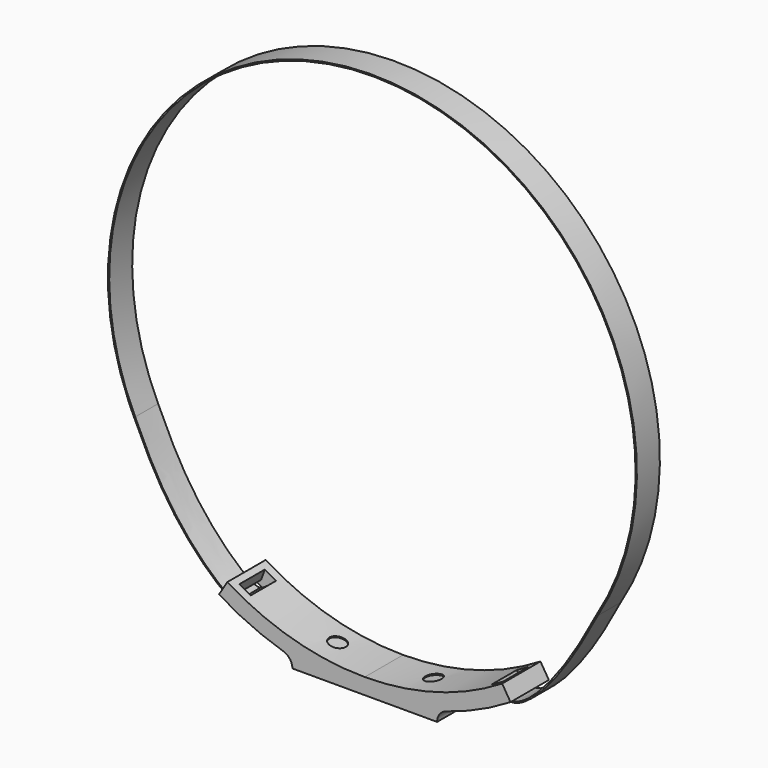
from build123d import *

# Parameters (mm, degrees)
F1_DEPTH     = 19.05
F3_D         = 6.5278
F3_DEPTH     = 101.6
F3_TIP       = 1.9611489744
F7_DEPTH     = 25.4
F9_DEPTH     = 25.4
F10_T1_DEPTH = 12.7
F11_T4_DEPTH = 19.05
F11_T9_DEPTH = 19.05
F13_START    = -3.81
F13_DEPTH    = 11.43


# Not quite as in the source:
# - a fillet or chamfer that OpenCascade refuses, or shapes differently, is made with other operations: its cross-section is extruded or revolved along the edge and cut away or added
# - ends of sketch curves that miss each other by under 0.0002 mm in the source are joined
# - the dataset's text gives a spline's control points without its knots; the knots are read off the source's solid


with BuildPart() as f1:
    # F0 (on Front) → F1 (new body)
    with BuildSketch(Plane.XZ):
        with BuildLine():
            Line((0, 0.9525), (28.7734375, 0.9525))
            Line((28.7734375, 0.9525), (28.7734375, 4.7648106998))
            ThreePointArc((28.7734375, 4.7648106998), (43.8235256978, 10.0149953703), (57.9615735284, 17.3760548981))
            Line((57.9615735284, 17.3760548981), (54.630448613, 22.7821724327))
            ThreePointArc((54.630448613, 22.7821724327), (28.390606608, 11.2471255737), (0, 7.3025))
            ThreePointArc((0, 7.3025), (-28.390606608, 11.2471255737), (-54.630448613, 22.7821724327))
            Line((-54.630448613, 22.7821724327), (-57.9615735284, 17.3760548981))
            ThreePointArc((-57.9615735284, 17.3760548981), (-43.8235256978, 10.0149953703), (-28.7734375, 4.7648106998))
            Line((-28.7734375, 4.7648106998), (-28.7734375, 0.9525))
            Line((-28.7734375, 0.9525), (0, 0.9525))
        make_face()
    extrude(amount=F1_DEPTH)

    # F3
    with Locations(Plane(origin=(0, 0, 0.9525), x_dir=(1, 0, 0), z_dir=(0, 0, -1))):
        with Locations((-19.05, 8.706397377), (19.05, 8.706397377)):
            Hole(F3_D / 2, depth=F3_DEPTH)
            with Locations((0, 0, -(F3_DEPTH + F3_TIP / 2))):  # 118° drill point
                Cone(0, F3_D / 2, F3_TIP, mode=Mode.SUBTRACT)

    # F6 (on face) → F7 (cut)
    with BuildSketch(Plane(origin=(0.9315005668, 0, 2.5592767734), x_dir=(0.9396926208, 0, -0.3420201433), z_dir=(0.3420201433, 0, 0.9396926208))):
        Polygon((-56.5877913126, -15.875), (-51.5077913126, -15.875), (-51.5077913126, -3.175), (-56.5877913126, -3.175), (-56.5877913126, -9.525), align=None)
    extrude(amount=-F7_DEPTH, mode=Mode.SUBTRACT)

    # F8 (on face) → F9 (cut)
    with BuildSketch(Plane(origin=(-0.9315005668, 0, 2.5592767734), x_dir=(0.9396926208, 0, 0.3420201433), z_dir=(-0.3420201433, 0, 0.9396926208))):
        Polygon((56.5877913126, -9.525), (56.5877913126, -3.175), (51.5077913126, -3.175), (51.5077913126, -15.875), (56.5877913126, -15.875), align=None)
    extrude(amount=-F9_DEPTH, mode=Mode.SUBTRACT)

    # F10: chamfer of 2.032 on 2 edges, made by hand

    # F10_s2 → F10_t1 (cut)
    with BuildSketch(Plane.XZ.offset(3.175)):
        with BuildLine():
            Line((-56.4802385277, 16.4064101357), (-53.8380025429, 17.3499641227))
            Line((-53.8380025429, 17.3499641227), (-53.7998134348, 17.3360644241))
            ThreePointArc((-53.7998134348, 17.3360644241), (-54.2182847726, 16.36929669), (-54.5779497805, 15.3811252023))
            Line((-54.5779497805, 15.3811252023), (-54.6362275834, 15.359697094))
            ThreePointArc((-54.6362275834, 15.359697094), (-55.5554397743, 15.8882458284), (-56.5009847135, 16.3714643867))
            Line((-56.5009847135, 16.3714643867), (-56.4802385277, 16.4064101357))
        make_face()
        with BuildLine():
            Line((56.4802385277, 16.4064101357), (53.8380025429, 17.3499641227))
            Line((53.8380025429, 17.3499641227), (53.7998134348, 17.3360644241))
            ThreePointArc((53.7998134348, 17.3360644241), (54.2182847726, 16.36929669), (54.5779497805, 15.3811252023))
            Line((54.5779497805, 15.3811252023), (54.6362275834, 15.359697094))
            ThreePointArc((54.6362275834, 15.359697094), (55.5554397743, 15.8882458284), (56.5009847135, 16.3714643867))
            Line((56.5009847135, 16.3714643867), (56.4802385277, 16.4064101357))
        make_face()
    extrude(amount=F10_T1_DEPTH, mode=Mode.SUBTRACT)

    # F11: fillet of radius 5.08 on 2 edges, made by hand


with BuildPart() as f11_tool2:
    # F11_s3 → F11_t4 (new body)
    with BuildSketch(Plane.XZ):
        with BuildLine():
            ThreePointArc((32.3653743132, 5.7991251695), (29.7689692978, 3.9624749409), (28.7734375, 0.9419585107))
            Line((28.7734375, 0.9419585107), (28.7734375, 4.7648106998))
            ThreePointArc((28.7734375, 4.7648106998), (30.5737800916, 5.266777394), (32.3653743132, 5.7991251695))
        make_face()
    extrude(amount=F11_T4_DEPTH)

    split(bisect_by=Plane.XY.offset(0.9525), keep=Keep.TOP)


with BuildPart() as f1_1:
    add(f1.part)

    # F11_t1: union F11_tool2
    add(f11_tool2.part)


with BuildPart() as f11_tool7:
    # F11_s8 → F11_t9 (new body)
    with BuildSketch(Plane.XZ):
        with BuildLine():
            ThreePointArc((-28.7734375, 0.9419585107), (-29.7689692978, 3.9624749409), (-32.3653743132, 5.7991251695))
            ThreePointArc((-32.3653743132, 5.7991251695), (-30.5737800916, 5.266777394), (-28.7734375, 4.7648106998))
            Line((-28.7734375, 4.7648106998), (-28.7734375, 0.9419585107))
        make_face()
    extrude(amount=F11_T9_DEPTH)

    split(bisect_by=Plane.XY.offset(0.9525), keep=Keep.TOP)


with BuildPart() as f1_2:
    add(f1_1.part)

    # F11_t6: union F11_tool7
    add(f11_tool7.part)


with BuildPart() as f13:
    # F12 (on face) → F13 (new body)
    with BuildSketch(Plane.XZ.offset(19.05).offset(F13_START)):
        with BuildLine():
            add(Edge.make_bspline(
                [(97.7812934658, 72.7565466816), (95.0915874954, 67.2526865805), (92.3916550741, 61.7538834708), (89.5893457762, 56.3831369507)],
                knots=[0, 0, 0, 0, 0.1467920374, 0.1467920374, 0.1467920374, 0.1467920374], degree=3))
            ThreePointArc((89.5893457762, 56.3831369507), (94.042337535, 64.3912185408), (97.7812934658, 72.7565466816))
        make_face()
        with BuildLine():
            add(Edge.make_bspline(
                [(89.112833025, 56.5680768855), (87.1535051538, 52.8143908139), (83.9230985786, 46.8814228282), (79.1843120961, 39.086281514), (75.0604811368, 32.9606078689), (70.6811123978, 27.195171834), (66.9878253233, 23.0075171537), (64.107119758, 20.212335288), (62.0108024209, 18.440572074), (60.0075643358, 17.04001445), (58.4439275603, 16.2205997367), (57.2751800485, 15.792809978), (56.447710407, 15.5904406243), (55.6612536188, 15.5025921765), (55.1398399584, 15.5086945326), (54.8758058385, 15.5283343935), (54.8530867048, 15.5301494973)],
                knots=[0.1472484928, 0.1472484928, 0.1472484928, 0.1472484928, 0.25, 0.3125, 0.375, 0.4375, 0.5, 0.53125, 0.5625, 0.59375, 0.625, 0.640625, 0.65625, 0.671875, 0.6875, 0.6889755322, 0.6889755322, 0.6889755322, 0.6889755322], degree=3))
            ThreePointArc((54.8530867048, 15.5301494973), (54.4873779941, 15.3219208334), (54.1208788351, 15.1150865908))
            add(Edge.make_bspline(
                [(89.5893457762, 56.3831369507), (85.3004601923, 48.1633029224), (75.0997889772, 30.3241377329), (60.7024662065, 14.841829536), (54.9116352389, 14.9693315987), (54.1208788351, 15.1150865908)],
                knots=[0.1467920374, 0.1467920374, 0.1467920374, 0.1467920374, 0.3714546946, 0.6528345101, 0.7032287333, 0.7032287333, 0.7032287333, 0.7032287333], degree=3))
            add(Edge.make_bspline(
                [(97.7812934658, 72.7565466816), (95.0915874954, 67.2526865805), (92.3916550741, 61.7538834708), (89.5893457762, 56.3831369507)],
                knots=[0, 0, 0, 0, 0.1467920374, 0.1467920374, 0.1467920374, 0.1467920374], degree=3))
            ThreePointArc((97.7812934658, 72.7565466816), (-1.0915815894, 216.5928342155), (-96.9570973239, 70.7349378707))
            add(Edge.make_bspline(
                [(-96.9570973239, 70.7349378707), (-96.2699684757, 69.1942721991), (-95.5817912633, 67.6542476227), (-94.885448022, 66.1155092588)],
                knots=[0, 0, 0, 0, 0.0480445963, 0.0480445963, 0.0480445963, 0.0480445963], degree=3))
            add(Edge.make_bspline(
                [(-94.885448022, 66.1155092588), (-90.0354933898, 55.3983645898), (-79.6735313167, 34.3533190654), (-57.5015516811, 13.5748962232), (-53.363721711, 14.4225193998), (-53.0698134343, 14.5320516363)],
                knots=[0.0480445963, 0.0480445963, 0.0480445963, 0.0480445963, 0.3826699627, 0.7089897606, 0.736391242, 0.736391242, 0.736391242, 0.736391242], degree=3))
            ThreePointArc((-53.0698134343, 14.5320516363), (-53.393256487, 14.7098774691), (-53.7161036897, 14.8887828038))
            add(Edge.make_bspline(
                [(-94.3249878412, 66.1093333744), (-93.2420344254, 63.7191576967), (-90.2940452977, 57.3422461891), (-85.9865677113, 49.0350531394), (-81.7231896657, 42.182614942), (-79.0480730962, 38.2922627791), (-76.9119458126, 35.3892927255), (-74.6283332446, 32.4968598043), (-71.4312912207, 28.7060070403), (-68.1062078289, 25.1211706689), (-64.8409274917, 21.9448539228), (-62.4700075431, 19.8182013503), (-60.2258045547, 17.9985331885), (-58.1591419069, 16.5377888749), (-56.6307697244, 15.663594476), (-55.5586001999, 15.1955970793), (-54.841625032, 14.9654820035), (-54.2243938183, 14.8583814899), (-53.8854699098, 14.8664131973), (-53.7237397991, 14.8877344036), (-53.7161036897, 14.8887828038)],
                knots=[0.0502911195, 0.0502911195, 0.0502911195, 0.0502911195, 0.125, 0.25, 0.3125, 0.34375, 0.375, 0.40625, 0.4375, 0.5, 0.53125, 0.5625, 0.59375, 0.625, 0.65625, 0.671875, 0.6875, 0.703125, 0.71875, 0.7195270393, 0.7195270393, 0.7195270393, 0.7195270393], degree=3))
            ThreePointArc((-94.3249878412, 66.1093333744), (5.4360404927, 215.9544649915), (89.112833025, 56.5680768855))
        make_face()
        with BuildLine():
            ThreePointArc((-96.9570973239, 70.7349378707), (-95.9490767615, 68.4127544207), (-94.885448022, 66.1155092588))
            add(Edge.make_bspline(
                [(-96.9570973239, 70.7349378707), (-96.2699684757, 69.1942721991), (-95.5817912633, 67.6542476227), (-94.885448022, 66.1155092588)],
                knots=[0, 0, 0, 0, 0.0480445963, 0.0480445963, 0.0480445963, 0.0480445963], degree=3))
        make_face()
        with BuildLine():
            ThreePointArc((54.1208788351, 15.1150865908), (54.4873779941, 15.3219208334), (54.8530867048, 15.5301494973))
            add(Edge.make_bspline(
                [(54.8530867048, 15.5301494973), (54.3946418593, 15.5667761121), (53.5078157419, 15.7423770413), (52.3566642919, 16.2141141425), (51.5780585738, 16.6933019848), (51.0985736249, 17.0606084253), (50.7663963395, 17.3340534027), (50.4215776233, 17.5963458323), (50.0198819854, 17.826521233), (49.6186110553, 17.9528293594), (49.2605213762, 17.995778311), (48.8912925087, 18.0008783124), (48.4528779364, 17.9543693016), (48.0888893332, 17.8811888286), (47.9275578829, 17.843704654)],
                knots=[0.6889755322, 0.6889755322, 0.6889755322, 0.6889755322, 0.71875, 0.75, 0.78125, 0.796875, 0.8125, 0.828125, 0.84375, 0.859375, 0.8671875, 0.875, 0.890625, 0.9024902953, 0.9024902953, 0.9024902953, 0.9024902953], degree=3))
            Line((47.9275578829, 17.843704654), (43.408251327, 16.2163214599))
            ThreePointArc((43.408251327, 16.2163214599), (0.7573475236, 6.7919969561), (-42.025488057, 15.5980441552))
            add(Edge.make_bspline(
                [(-53.7161036897, 14.8887828038), (-53.5701900202, 14.9088160324), (-53.2900470116, 14.978644905), (-52.8907566688, 15.1599576115), (-52.4872099402, 15.4134020086), (-52.0719397585, 15.7169129221), (-51.6290014012, 16.0446951453), (-51.1389043543, 16.3660024589), (-50.6717898209, 16.5990811154), (-50.2574791706, 16.7415137761), (-49.8303192702, 16.8502861072), (-49.2700265762, 16.9308447204), (-48.3261113032, 16.9591345215), (-47.0637204526, 16.8365561474), (-45.4429828571, 16.5128060575), (-43.7499737798, 16.0779855487), (-42.5992478875, 15.7563509731), (-42.025488057, 15.5980441552)],
                knots=[0.7195270393, 0.7195270393, 0.7195270393, 0.7195270393, 0.734375, 0.75, 0.765625, 0.78125, 0.796875, 0.8125, 0.828125, 0.8359375, 0.84375, 0.859375, 0.875, 0.90625, 0.9375, 0.96875, 0.9999988144, 0.9999988144, 0.9999988144, 0.9999988144], degree=3))
            ThreePointArc((-53.7161036897, 14.8887828038), (-53.393256487, 14.7098774691), (-53.0698134343, 14.5320516363))
            add(Edge.make_bspline(
                [(-53.0698134343, 14.5320516363), (-52.0681969868, 14.905328942), (-50.1139300611, 17.3973337636), (-45.2919867438, 15.9723255411), (-42.1605369582, 15.1083240322)],
                knots=[0.736391242, 0.736391242, 0.736391242, 0.736391242, 0.82977335, 1, 1, 1, 1], degree=3))
            ThreePointArc((-42.1605369582, 15.1083240322), (0.7365801988, 6.2890797722), (43.5059395829, 15.7084018061))
            add(Edge.make_bspline(
                [(54.1208788351, 15.1150865908), (52.8236146579, 15.354202871), (50.7619859651, 16.4827791328), (49.3882914075, 18.1764224999), (45.8043035123, 16.6232383684), (43.5059395829, 15.7084018061)],
                knots=[0.7032287333, 0.7032287333, 0.7032287333, 0.7032287333, 0.7859022599, 0.8642986928, 1, 1, 1, 1], degree=3))
        make_face()
    extrude(amount=-F13_DEPTH)


solid = Compound([f1_2.part, f13.part])
